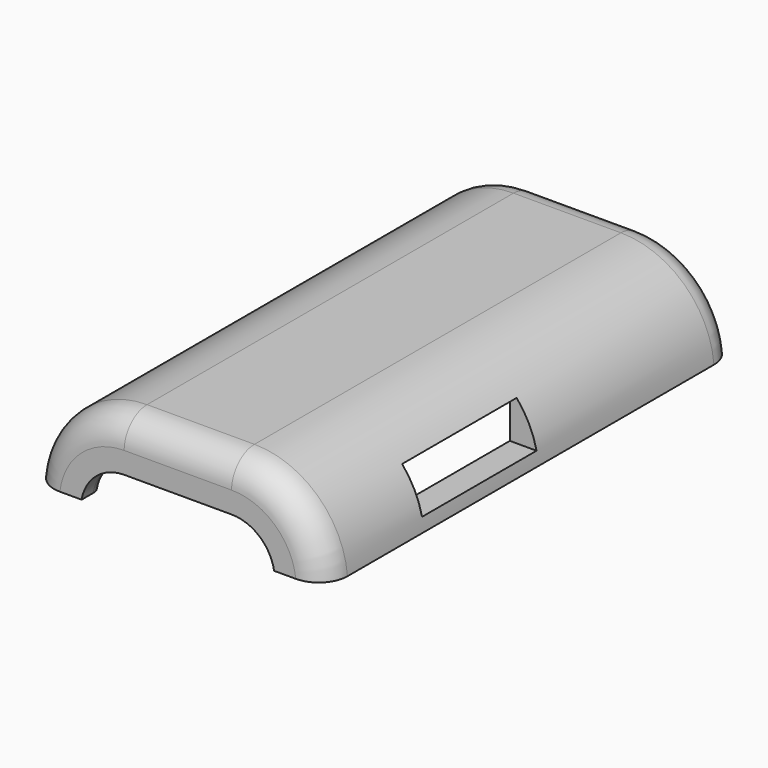
from build123d import *

# Parameters (mm, degrees)
F1_W           = 20.5
F1_H           = 36
F2_DEPTH       = 6
F0_W           = 16.5
F0_H           = 32
F3_DEPTH       = 4
F4_T1_DEPTH    = 68.4886593371
F5_R           = 2
F7_DEPTH       = 25
F7_DEPTH_BACK  = 20.4
F8_R           = 1
F9_W           = 10
F9_H           = 2.8
F10_DEPTH      = 25
F10_DEPTH_BACK = 25


# Not quite as in the source:
# - a fillet or chamfer that OpenCascade refuses, or shapes differently, is made with other operations: its cross-section is extruded or revolved along the edge and cut away or added


with BuildPart() as f2:
    # F1 (on Top) → F2 (new body)
    with BuildSketch(Plane.XY):
        with Locations((0.1103486419, -0.6806470305)):
            Rectangle(F1_W, F1_H)
    extrude(amount=F2_DEPTH)

    # F0 (on Top) → F3 (cut)
    with BuildSketch(Plane.XY):
        with Locations((0.1103486419, -0.6806470305)):
            Rectangle(F0_W, F0_H)
    extrude(amount=F3_DEPTH, mode=Mode.SUBTRACT)

    # F4: fillet of radius 6.5183766184 on 2 edges, made by hand

    # F4_s2 → F4_t1 (cut)
    with BuildSketch(Plane.XZ.offset(-33.5636826381)):
        with BuildLine():
            ThreePointArc((10.3603486419, 0), (8.2847350288, 4.270579832), (3.8626167745, 6))
            Line((3.8626167745, 6), (10.3603486419, 6))
            Line((10.3603486419, 6), (10.3603486419, 0))
        make_face()
        with BuildLine():
            ThreePointArc((-10.1396513581, 0), (-8.064037745, 4.270579832), (-3.6419194907, 6))
            Line((-3.6419194907, 6), (-10.1396513581, 6))
            Line((-10.1396513581, 6), (-10.1396513581, 0))
        make_face()
    extrude(amount=F4_T1_DEPTH, mode=Mode.SUBTRACT)

    # F5
    f5_edges = [f2.edges().sort_by_distance(p)[0] for p in [
        (0.110349, 17.319353, 6),
        (8.284735, 17.319353, 4.27058),
        (-8.064038, -18.680647, 4.27058),
        (-8.064038, 17.319353, 4.27058),
        (0.110349, -18.680647, 6),
        (8.284735, -18.680647, 4.27058),
    ]]
    fillet(f5_edges, radius=F5_R)

    # F6 (on Front) → F7 (cut, two sides)
    with BuildSketch(Plane.XZ) as f7_sk:
        with BuildLine():
            ThreePointArc((6.8361471832, 0), (5.8050304207, 1.791953799), (3.8626167745, 2.5))
            Line((3.8626167745, 2.5), (-3.6419194907, 2.5))
            ThreePointArc((-3.6419194907, 2.5), (-5.5843331369, 1.791953799), (-6.6154498995, 0))
            Line((-6.6154498995, 0), (6.8361471832, 0))
        make_face()
    extrude(amount=-F7_DEPTH, mode=Mode.SUBTRACT)
    extrude(f7_sk.sketch, amount=F7_DEPTH_BACK, mode=Mode.SUBTRACT)

    # F8
    f8_edges = [f2.edges().sort_by_distance(p)[0] for p in [
        (-5.584333, 15.319353, 1.791954),
        (0.110349, -16.680647, 2.5),
        (5.80503, 15.319353, 1.791954),
        (0.110349, 15.319353, 2.5),
        (5.80503, -16.680647, 1.791954),
        (-5.584333, -16.680647, 1.791954),
    ]]
    fillet(f8_edges, radius=F8_R)

    # F9 (on Right) → F10 (cut, two sides)
    with BuildSketch(Plane.YZ) as f10_sk:
        with Locations((-5, 2.2957557753)):
            Rectangle(F9_W, F9_H)
    extrude(amount=-F10_DEPTH, mode=Mode.SUBTRACT)
    extrude(f10_sk.sketch, amount=F10_DEPTH_BACK, mode=Mode.SUBTRACT)


solid = f2.part
